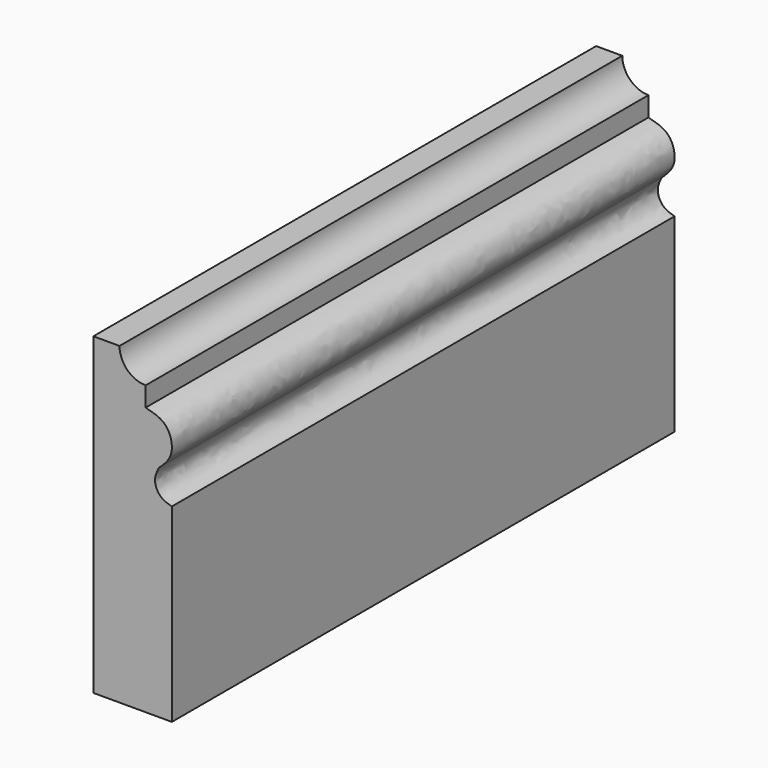
from build123d import *

# Parameters (mm, degrees)
F1_DEPTH = 152.4


# Not quite as in the source:
# - ends of sketch curves that miss each other by under 0.0002 mm in the source are joined
# - the dataset's text gives a spline's control points without its knots; the knots are read off the source's solid


with BuildPart() as f1:
    # F0 (on Front) → F1 (new body)
    with BuildSketch(Plane.XZ):
        with BuildLine():
            Line((9.5127572, -38.0712472), (9.5127572, 7.931531))
            add(Edge.make_bspline(
                [(6.3401448, 15.1268176), (5.8891424, 14.1770608), (4.9154588, 12.1265696), (6.532499, 8.7763096), (8.6041992, 8.1890616), (9.5127572, 7.931531)],
                knots=[0, 0, 0, 0, 0.120135, 0.259368, 0.368128, 0.368128, 0.368128, 0.368128], degree=3))
            add(Edge.make_bspline(
                [(3.1675578, 26.9671546), (4.9711102, 26.507059), (8.7999316, 25.5303274), (10.3429562, 18.8598302), (7.5847956, 16.2875722), (6.3401448, 15.1268176)],
                knots=[0, 0, 0, 0, 0.207787, 0.441117, 0.632993, 0.632993, 0.632993, 0.632993], degree=3))
            Line((3.1675578, 26.9671546), (3.1675578, 31.7260478))
            ThreePointArc((3.1675578, 31.7260478), (-1.3191757237, 33.5845390763), (-3.1776416, 38.0712726))
            Line((-3.1776416, 38.0712726), (-9.5228664, 38.0712726))
            Line((-9.5228664, 38.0712726), (-9.5228664, -38.0712472))
            Line((-9.5228664, -38.0712472), (9.5127572, -38.0712472))
        make_face()
    extrude(amount=F1_DEPTH)


solid = f1.part
